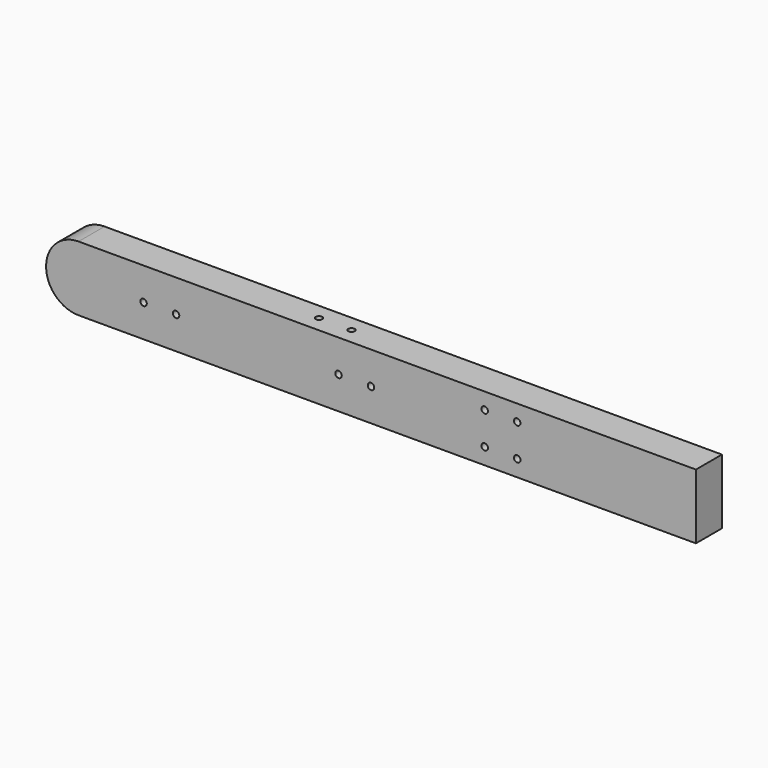
from build123d import *

# Parameters (mm, degrees)
F0_W     = 1000
F0_H     = 100
F1_DEPTH = 50
F3_R     = 5
F4_DEPTH = 25
F2_R     = 5
F5_DEPTH = 50
F6_R     = 5
F7_DEPTH = 50
F8_R     = 49.99999


# Not quite as in the source:
# - a fillet or chamfer is up to 0.001 mm smaller than in the source, because OpenCascade refuses the exact size


with BuildPart() as f1:
    # F0 (on Front) → F1 (new body)
    with BuildSketch(Plane.XZ):
        Rectangle(F0_W, F0_H)
    extrude(amount=F1_DEPTH)

    # F3 (on face) → F4 (cut)
    with BuildSketch(Plane.XY.offset(50)):
        with Locations((-100, -25)):
            Circle(F3_R)
        with Locations((-50, -25)):
            Circle(F3_R)
    extrude(amount=-F4_DEPTH, mode=Mode.SUBTRACT)

    # F2 (on face) → F5 (cut)
    with BuildSketch(Plane.XZ.offset(50)):
        with Locations((-50, 0)):
            Circle(F2_R)
        Circle(F2_R)
        with Locations((-350, 0)):
            Circle(F2_R)
        with Locations((-300, 0)):
            Circle(F2_R)
    extrude(amount=-F5_DEPTH, mode=Mode.SUBTRACT)

    # F6 (on face) → F7 (cut)
    with BuildSketch(Plane(origin=(0, 0, 0), x_dir=(-1, 0, 0), z_dir=(0, 1, 0))):
        with Locations((-225, -25)):
            Circle(F6_R)
        with Locations((-175, -25)):
            Circle(F6_R)
        with Locations((-225, 25)):
            Circle(F6_R)
        with Locations((-175, 25)):
            Circle(F6_R)
    extrude(amount=-F7_DEPTH, mode=Mode.SUBTRACT)

    # F8 (radius 50 in the source; OpenCascade refuses exactly that, so slightly less here)
    f8_edges = [f1.edges().sort_by_distance(p)[0] for p in [
        (-500, -25, 50),
        (-500, -25, -50),
    ]]
    fillet(f8_edges, radius=F8_R)


solid = f1.part
